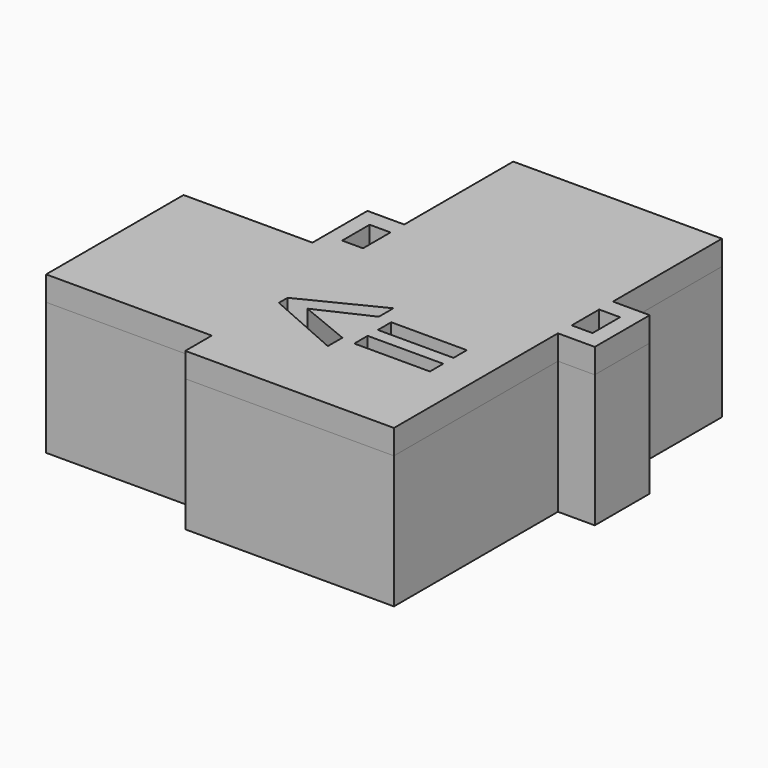
from build123d import *

# Parameters (mm, degrees)
F1_DEPTH      = 9.2
F2_DEPTH      = 1
F3_DEPTH      = 9.8
F5_DEPTH      = 0.6
F7_DEPTH      = 2
F8_W          = 11
F8_H          = 0.8
F8_H_2        = 2.7
F9_DEPTH      = 1.5000002086
F10_TEXT_SIZE = 12.7033511591
F11_DEPTH     = 2
F12_DEPTH     = 1


# Not quite as in the source:
# - Text() gives the source's letters only with a copy of the font that has no kerning and outlines rounded to 1/6400 em; it was checked with that copy


with BuildPart() as f1:
    # F0 (on Top) → F1 (new body)
    with BuildSketch(Plane.XY):
        Polygon((-8.5000002086, 1.4000002086), (-8.5000002086, 2.086e-07), (-11.5000002086, 2.086e-07), (-22.0000002086, 2.086e-07), (-22.0000002086, -14.0000002086), (-8.5000002086, -14.0000002086), (-8.5000002086, -16.7000002086), (8.5000002086, -16.7000002086), (8.5000002086, 2.086e-07), (8.5000002086, 1.4000002086), (8.5000002086, 4.2000002086), (8.5000002086, 5.6000002086), (8.5000002086, 16.7000002086), (-8.5000002086, 16.7000002086), (-8.5000002086, 5.6000002086), (-8.5000002086, 4.2000002086), align=None)
        Polygon((-21.2500000857, -0.7499999143), (-7.7500000857, -0.7499999143), (-7.7500000857, 15.9500000857), (7.7500000857, 15.9500000857), (7.7500000857, -15.9500000857), (-7.7500000857, -15.9500000857), (-7.7500000857, -13.2500000857), (-21.2500000857, -13.2500000857), align=None, mode=Mode.SUBTRACT)
        Polygon((-11.5000002086, 2.086e-07), (-8.5000002086, 2.086e-07), (-8.5000002086, 1.4000002086), (-10.2000002086, 1.4000002086), (-10.2000002086, 4.2000002086), (-8.5000002086, 4.2000002086), (-8.5000002086, 5.6000002086), (-11.5000002086, 5.6000002086), align=None)
        Polygon((11.5000002086, 5.6000002086), (8.5000002086, 5.6000002086), (8.5000002086, 4.2000002086), (10.2000002086, 4.2000002086), (10.2000002086, 1.4000002086), (8.5000002086, 1.4000002086), (8.5000002086, 2.086e-07), (11.5000002086, 2.086e-07), align=None)
        Polygon((-7.7500000857, 15.9500000857), (-7.7500000857, -0.7499999143), (-21.2500000857, -0.7499999143), (-21.2500000857, -13.2500000857), (-7.7500000857, -13.2500000857), (-7.7500000857, -15.9500000857), (7.7500000857, -15.9500000857), (7.7500000857, 15.9500000857), align=None)
        Polygon((7, 15.2), (7, -15.2), (-7, -15.2), (-7, -12.5), (-20.5, -12.5), (-20.5, -1.5), (-7, -1.5), (-7, 15.2), align=None, mode=Mode.SUBTRACT)
    extrude(amount=F1_DEPTH)

    # F0 (on Top) → F2 (join)
    with BuildSketch(Plane.XY):
        Polygon((-8.5000002086, 1.4000002086), (-8.5000002086, 2.086e-07), (-11.5000002086, 2.086e-07), (-22.0000002086, 2.086e-07), (-22.0000002086, -14.0000002086), (-8.5000002086, -14.0000002086), (-8.5000002086, -16.7000002086), (8.5000002086, -16.7000002086), (8.5000002086, 2.086e-07), (8.5000002086, 1.4000002086), (8.5000002086, 4.2000002086), (8.5000002086, 5.6000002086), (8.5000002086, 16.7000002086), (-8.5000002086, 16.7000002086), (-8.5000002086, 5.6000002086), (-8.5000002086, 4.2000002086), align=None)
        Polygon((-21.2500000857, -0.7499999143), (-7.7500000857, -0.7499999143), (-7.7500000857, 15.9500000857), (7.7500000857, 15.9500000857), (7.7500000857, -15.9500000857), (-7.7500000857, -15.9500000857), (-7.7500000857, -13.2500000857), (-21.2500000857, -13.2500000857), align=None, mode=Mode.SUBTRACT)
        Polygon((-7.7500000857, 15.9500000857), (-7.7500000857, -0.7499999143), (-21.2500000857, -0.7499999143), (-21.2500000857, -13.2500000857), (-7.7500000857, -13.2500000857), (-7.7500000857, -15.9500000857), (7.7500000857, -15.9500000857), (7.7500000857, 15.9500000857), align=None)
        Polygon((7, 15.2), (7, -15.2), (-7, -15.2), (-7, -12.5), (-20.5, -12.5), (-20.5, -1.5), (-7, -1.5), (-7, 15.2), align=None, mode=Mode.SUBTRACT)
        Polygon((-7, -15.2), (7, -15.2), (7, 15.2), (-7, 15.2), (-7, -1.5), (-20.5, -1.5), (-20.5, -12.5), (-7, -12.5), align=None)
    extrude(amount=-F2_DEPTH)

    # F0 (on Top) → F3 (join)
    with BuildSketch(Plane.XY):
        Polygon((-8.5000002086, 1.4000002086), (-8.5000002086, 2.086e-07), (-11.5000002086, 2.086e-07), (-22.0000002086, 2.086e-07), (-22.0000002086, -14.0000002086), (-8.5000002086, -14.0000002086), (-8.5000002086, -16.7000002086), (8.5000002086, -16.7000002086), (8.5000002086, 2.086e-07), (8.5000002086, 1.4000002086), (8.5000002086, 4.2000002086), (8.5000002086, 5.6000002086), (8.5000002086, 16.7000002086), (-8.5000002086, 16.7000002086), (-8.5000002086, 5.6000002086), (-8.5000002086, 4.2000002086), align=None)
        Polygon((-21.2500000857, -0.7499999143), (-7.7500000857, -0.7499999143), (-7.7500000857, 15.9500000857), (7.7500000857, 15.9500000857), (7.7500000857, -15.9500000857), (-7.7500000857, -15.9500000857), (-7.7500000857, -13.2500000857), (-21.2500000857, -13.2500000857), align=None, mode=Mode.SUBTRACT)
        Polygon((11.5000002086, 5.6000002086), (8.5000002086, 5.6000002086), (8.5000002086, 4.2000002086), (10.2000002086, 4.2000002086), (10.2000002086, 1.4000002086), (8.5000002086, 1.4000002086), (8.5000002086, 2.086e-07), (11.5000002086, 2.086e-07), align=None)
        Polygon((-11.5000002086, 2.086e-07), (-8.5000002086, 2.086e-07), (-8.5000002086, 1.4000002086), (-10.2000002086, 1.4000002086), (-10.2000002086, 4.2000002086), (-8.5000002086, 4.2000002086), (-8.5000002086, 5.6000002086), (-11.5000002086, 5.6000002086), align=None)
    extrude(amount=F3_DEPTH)

    # F8 (on face) → F9 (cut, through all)
    with BuildSketch(Plane(origin=(-22.0000002086, 0, 0), x_dir=(0, -1, 0), z_dir=(-1, 0, 0))):
        with Locations((7, 9.4)):
            Rectangle(F8_W, F8_H)
        with Locations((7, 7.65)):
            Rectangle(F8_W, F8_H_2)
    extrude(amount=-F9_DEPTH, mode=Mode.SUBTRACT)

    # F0 (on Top) → F12 (join, through all)
    with BuildSketch(Plane.XY):
        Polygon((-11.5000002086, 2.086e-07), (-8.5000002086, 2.086e-07), (-8.5000002086, 1.4000002086), (-10.2000002086, 1.4000002086), (-10.2000002086, 4.2000002086), (-8.5000002086, 4.2000002086), (-8.5000002086, 5.6000002086), (-11.5000002086, 5.6000002086), align=None)
        Polygon((11.5000002086, 5.6000002086), (8.5000002086, 5.6000002086), (8.5000002086, 4.2000002086), (10.2000002086, 4.2000002086), (10.2000002086, 1.4000002086), (8.5000002086, 1.4000002086), (8.5000002086, 2.086e-07), (11.5000002086, 2.086e-07), align=None)
    extrude(amount=-F12_DEPTH)


with BuildPart() as f5:
    # F4 (on face) → F5 (new body, through all)
    with BuildSketch(Plane.XY.offset(9.2)):
        Polygon((-7.7500000857, 15.9500000857), (-7.7500000857, -0.7499999143), (-21.2500000857, -0.7499999143), (-21.2500000857, -13.2500000857), (-7.7500000857, -13.2500000857), (-7.7500000857, -15.9500000857), (7.7500000857, -15.9500000857), (7.7500000857, 15.9500000857), align=None)
        Polygon((-20.5, -1.5), (-7, -1.5), (-7, 15.2), (7, 15.2), (7, -15.2), (-7, -15.2), (-7, -12.5), (-20.5, -12.5), align=None, mode=Mode.SUBTRACT)
    extrude(amount=F5_DEPTH)

    # F6 (on face) → F7 (join)
    with BuildSketch(Plane.XY.offset(9.8)):
        Polygon((-8.5000002086, 1.4000002086), (-8.5000002086, 2.086e-07), (-11.5000002086, 2.086e-07), (-22.0000002086, 2.086e-07), (-22.0000002086, -14.0000002086), (-8.5000002086, -14.0000002086), (-8.5000002086, -16.7000002086), (8.5000002086, -16.7000002086), (8.5000002086, 2.086e-07), (8.5000002086, 1.4000002086), (8.5000002086, 4.2000002086), (8.5000002086, 5.6000002086), (8.5000002086, 16.7000002086), (-8.5000002086, 16.7000002086), (-8.5000002086, 5.6000002086), (-8.5000002086, 4.2000002086), align=None)
        Polygon((-11.5000002086, 2.086e-07), (-8.5000002086, 2.086e-07), (-8.5000002086, 1.4000002086), (-10.2000002086, 1.4000002086), (-10.2000002086, 4.2000002086), (-8.5000002086, 4.2000002086), (-8.5000002086, 5.6000002086), (-11.5000002086, 5.6000002086), align=None)
        Polygon((11.5000002086, 5.6000002086), (8.5000002086, 5.6000002086), (8.5000002086, 4.2000002086), (10.2000002086, 4.2000002086), (10.2000002086, 1.4000002086), (8.5000002086, 1.4000002086), (8.5000002086, 2.086e-07), (11.5000002086, 2.086e-07), align=None)
    extrude(amount=F7_DEPTH)

    # F10 (on face) → F11 (cut, through all)
    with BuildSketch(Plane.XY.offset(11.8)):
        with Locations((-8.5311704315, -11.785951443)):
            Text('<=', F10_TEXT_SIZE, font='Open Sans', font_style=FontStyle.BOLD, text_align=(TextAlign.LEFT, TextAlign.BOTTOM))
    extrude(amount=-F11_DEPTH, mode=Mode.SUBTRACT)


solid = Compound([f1.part, f5.part])
